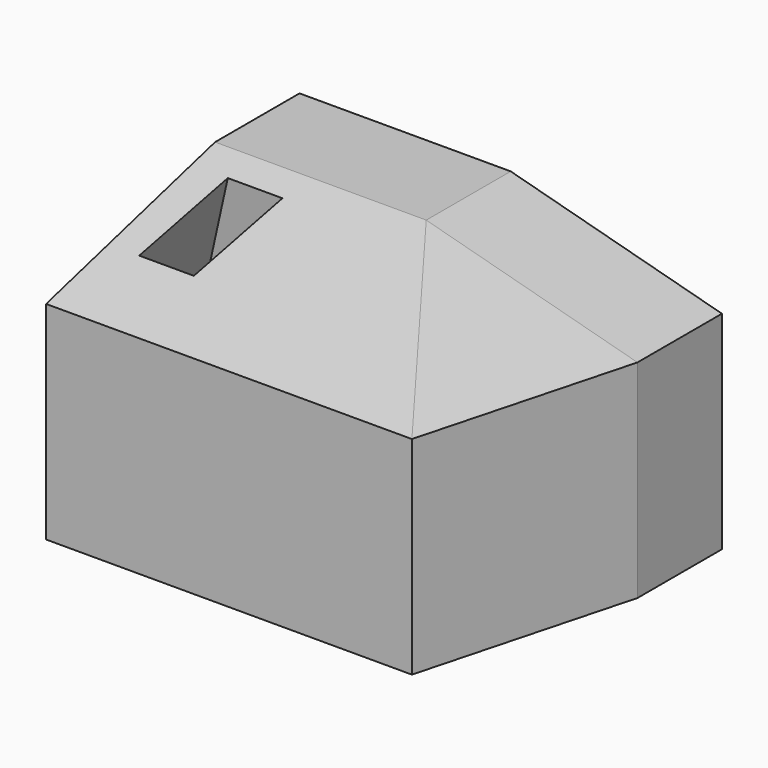
from build123d import *

# Parameters (mm, degrees)
F0_W        = 80
F0_H        = 50
F1_DEPTH    = 60
F2_T1_DEPTH = 14.4048552446
F2_T3_DEPTH = 287.737725616
F2_T5_DEPTH = 267.737725616
F2_T7_DEPTH = 257.737725616
F3_W        = 10
F3_H        = 20
F4_DEPTH    = 59.8932080195


# Not quite as in the source:
# - a fillet or chamfer that OpenCascade refuses, or shapes differently, is made with other operations: its cross-section is extruded or revolved along the edge and cut away or added


with BuildPart() as f1:
    # F0 (on Front) → F1 (new body)
    with BuildSketch(Plane.XZ):
        with Locations((40, 25)):
            Rectangle(F0_W, F0_H)
    extrude(amount=F1_DEPTH)

    # F2: chamfer of 40 x 10.7179676972 on 3 edges, made by hand

    # F2_s2 → F2_t1 (cut)
    with BuildSketch(Plane(origin=(15.4641016151, -4.1435935394, 57.7128129211), x_dir=(0.2588190451, 0.9659258263, 0), z_dir=(0.2581988897, -0.069184184, 0.963611375))):
        Polygon((1.3870070824, -68.9498200994), (-8.9657547217, -28.8537460449), (-40.024040134, -68.9498200994), align=None)
    extrude(amount=F2_T1_DEPTH, mode=Mode.SUBTRACT)

    # F2_s4 → F2_t3 (cut)
    with BuildSketch(Plane.YZ.offset(-103.868862808)):
        Polygon((-20, 50), (-60, 39.2820323028), (-60, 50), align=None)
    extrude(amount=F2_T3_DEPTH, mode=Mode.SUBTRACT)

    # F2_s6 → F2_t5 (cut)
    with BuildSketch(Plane.XZ.offset(-103.868862808)):
        Polygon((80, 39.2820323028), (40, 50), (80, 50), align=None)
    extrude(amount=F2_T5_DEPTH, mode=Mode.SUBTRACT)

    # F2_s8 → F2_t7 (cut)
    with BuildSketch(Plane.XY.offset(-103.868862808)):
        Polygon((80, -20), (69.2820323028, -60), (80, -60), align=None)
    extrude(amount=F2_T7_DEPTH, mode=Mode.SUBTRACT)

    # F3 (on face) → F4 (cut, through all)
    with BuildSketch(Plane(origin=(15.4641016151, -4.1435935394, 57.7128129211), x_dir=(0.9660917831, 0.0184902509, -0.2575359728), z_dir=(0.2581988897, -0.069184184, 0.963611375))):
        with Locations((-1.3299316186, -32.0328700794)):
            Rectangle(F3_W, F3_H)
    extrude(amount=-F4_DEPTH, mode=Mode.SUBTRACT)


solid = f1.part
